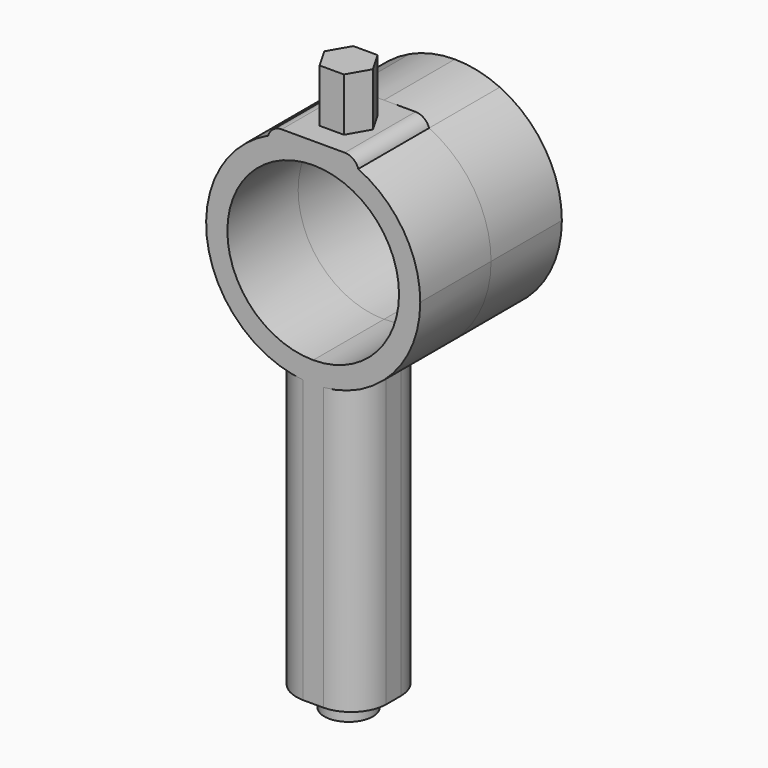
from build123d import *

# Parameters (mm, degrees)
F1_DEPTH     = 12.5
F2_DEPTH     = 12.5
F3_DEPTH     = 12.5
F6_DEPTH     = 7.5
F5_R         = 3.429
F7_DEPTH     = 3
F8_T4_DEPTH  = 66.159380005
F8_S5_R      = 15.125
F8_T6_DEPTH  = 35
F8_T10_DEPTH = 66.159380005
F8_S11_R     = 15.125
F8_T12_DEPTH = 35
F8_T16_DEPTH = 66.159380005
F8_S17_R     = 15.125
F8_T18_DEPTH = 35
F8_T22_DEPTH = 66.159380005
F8_S23_R     = 15.125
F8_T24_DEPTH = 35
F9_T1_DEPTH  = 22.0465191056


# Not quite as in the source:
# - a fillet or chamfer that OpenCascade refuses, or shapes differently, is made with other operations: its cross-section is extruded or revolved along the edge and cut away or added


with BuildPart() as f1:
    # F0 (on Front) → F1 (new body, symmetric)
    with BuildSketch(Plane.XZ):
        with BuildLine():
            Line((-6.3651329838, -12.125), (-6.3651329838, -13.7204485021))
            ThreePointArc((-6.3651329838, -13.7204485021), (0, -15.125), (6.3651329838, -13.7204485021))
            Line((6.3651329838, -13.7204485021), (6.3651329838, -12.125))
            Line((6.3651329838, -12.125), (0, -12.125))
            Line((0, -12.125), (-6.3651329838, -12.125))
        make_face()
        with BuildLine():
            ThreePointArc((6.3651329838, 13.7204485021), (3.2591288258, 14.7696887001), (0, 15.125))
            ThreePointArc((0, 15.125), (-3.2591288258, 14.7696887001), (-6.3651329838, 13.7204485021))
            Line((-6.3651329838, 13.7204485021), (-6.3651329838, 12.125))
            Line((-6.3651329838, 12.125), (0, 12.125))
            Line((0, 12.125), (6.3651329838, 12.125))
            Line((6.3651329838, 12.125), (6.3651329838, 13.7204485021))
        make_face()
        with BuildLine():
            ThreePointArc((15.125, 0), (12.7482991293, 8.1391949424), (6.3651329838, 13.7204485021))
            Line((6.3651329838, 13.7204485021), (6.3651329838, 12.125))
            Line((6.3651329838, 12.125), (0, 12.125))
            ThreePointArc((0, 12.125), (8.5736697219, 8.5736697219), (12.125, 0))
            ThreePointArc((12.125, 0), (8.5736697219, -8.5736697219), (0, -12.125))
            Line((0, -12.125), (6.3651329838, -12.125))
            Line((6.3651329838, -12.125), (6.3651329838, -13.7204485021))
            ThreePointArc((6.3651329838, -13.7204485021), (12.7482991293, -8.1391949424), (15.125, 0))
        make_face()
        with BuildLine():
            Line((-6.3651329838, 12.125), (-6.3651329838, 13.7204485021))
            ThreePointArc((-6.3651329838, 13.7204485021), (-15.125, 0), (-6.3651329838, -13.7204485021))
            Line((-6.3651329838, -13.7204485021), (-6.3651329838, -12.125))
            Line((-6.3651329838, -12.125), (0, -12.125))
            ThreePointArc((0, -12.125), (-12.125, 0), (0, 12.125))
            Line((0, 12.125), (-6.3651329838, 12.125))
        make_face()
    extrude(amount=F1_DEPTH, both=True)

    # F0 (on Front) → F2 (join, through all)
    with BuildSketch(Plane.XZ):
        with BuildLine():
            ThreePointArc((6.3651329838, -13.7204485021), (0, -15.125), (-6.3651329838, -13.7204485021))
            Line((-6.3651329838, -13.7204485021), (-6.3651329838, -54.875))
            Line((-6.3651329838, -54.875), (6.3651329838, -54.875))
            Line((6.3651329838, -54.875), (6.3651329838, -13.7204485021))
        make_face()
    extrude(amount=F2_DEPTH)

    # F0 (on Front) → F3 (join, through all)
    with BuildSketch(Plane.XZ):
        with BuildLine():
            Line((6.3651329838, 15.125), (0, 15.125))
            ThreePointArc((0, 15.125), (3.2591288258, 14.7696887001), (6.3651329838, 13.7204485021))
            Line((6.3651329838, 13.7204485021), (6.3651329838, 15.125))
        make_face()
        with BuildLine():
            Line((0, 15.125), (-6.3651329838, 15.125))
            Line((-6.3651329838, 15.125), (-6.3651329838, 13.7204485021))
            ThreePointArc((-6.3651329838, 13.7204485021), (-3.2591288258, 14.7696887001), (0, 15.125))
        make_face()
    extrude(amount=F3_DEPTH)

    # F4 (on face) → F6 (join)
    with BuildSketch(Plane.XY.offset(15.125)):
        Polygon((1.7145000001, -9.2196011096), (3.4290000001, -6.25), (1.7144999999, -3.2803988905), (-1.7145, -3.2803988907), (-3.4289999999, -6.25), (-1.7145000001, -9.2196011096), align=None)
    extrude(amount=F6_DEPTH)

    # F5 (on face) → F7 (join)
    with BuildSketch(Plane(origin=(0, 0, -54.875), x_dir=(1, 0, 0), z_dir=(0, 0, -1))):
        with Locations((0, 6.2500000003)):
            Circle(F5_R)
    extrude(amount=F7_DEPTH)

    # F8: fillet of radius 5 on 6 edges, made by hand


with BuildPart() as f8_tool2:
    # F8_s3 → F8_t4 (new body)
    with BuildSketch(Plane.XY.offset(-67.3774142536)):
        with BuildLine():
            ThreePointArc((1.3641672983, 0.0004), (4.9006668897, -1.4644660941), (6.3655329838, -5.0009656854))
            Line((6.3655329838, -5.0009656854), (6.8656695523, -5.0009656854))
            ThreePointArc((6.8656695523, -5.0009656854), (6.8652695523, -2.5004828427), (6.8652695523, 0))
            Line((6.8652695523, 0), (6.3651329838, 0.5001365685))
            ThreePointArc((6.3651329838, 0.5001365685), (3.8646501411, 0.5001365685), (1.3641672983, 0.5005365685))
            Line((1.3641672983, 0.5005365685), (1.3641672983, 0.0004))
        make_face()
    extrude(amount=F8_T4_DEPTH)

    # F8_s5 → F8_t6 (cut, symmetric)
    with BuildSketch(Plane.XZ.offset(2.3)):
        Circle(F8_S5_R)
    extrude(amount=F8_T6_DEPTH, both=True, mode=Mode.SUBTRACT)


with BuildPart() as f1_1:
    add(f1.part)

    # F8_t1: cut F8_tool2
    add(f8_tool2.part, mode=Mode.SUBTRACT)


with BuildPart() as f8_tool8:
    # F8_s9 → F8_t10 (new body)
    with BuildSketch(Plane.XY.offset(-1.2180342485)):
        with BuildLine():
            ThreePointArc((-6.3655329838, -5.0009656854), (-4.9006668897, -1.4644660941), (-1.3641672983, 0.0004))
            Line((-1.3641672983, 0.0004), (-1.3641672983, 0.5005365685))
            ThreePointArc((-1.3641672983, 0.5005365685), (-3.8646501411, 0.5001365685), (-6.3651329838, 0.5001365685))
            Line((-6.3651329838, 0.5001365685), (-6.8652695523, 0))
            ThreePointArc((-6.8652695523, 0), (-6.8652695523, -2.5004828427), (-6.8656695523, -5.0009656854))
            Line((-6.8656695523, -5.0009656854), (-6.3655329838, -5.0009656854))
        make_face()
    extrude(amount=-F8_T10_DEPTH)

    # F8_s11 → F8_t12 (cut, symmetric)
    with BuildSketch(Plane.XZ.offset(2.3)):
        Circle(F8_S11_R)
    extrude(amount=F8_T12_DEPTH, both=True, mode=Mode.SUBTRACT)


with BuildPart() as f1_2:
    add(f1_1.part)

    # F8_t7: cut F8_tool8
    add(f8_tool8.part, mode=Mode.SUBTRACT)


with BuildPart() as f8_tool14:
    # F8_s15 → F8_t16 (new body)
    with BuildSketch(Plane.XY.offset(-67.3774142536)):
        with BuildLine():
            ThreePointArc((1.3641672983, -12.5004), (4.9006668897, -11.0355339059), (6.3655329838, -7.4990343146))
            Line((6.3655329838, -7.4990343146), (6.8656695523, -7.4990343146))
            ThreePointArc((6.8656695523, -7.4990343146), (6.8652695523, -9.9995171573), (6.8652695523, -12.5))
            Line((6.8652695523, -12.5), (6.3651329838, -13.0001365685))
            ThreePointArc((6.3651329838, -13.0001365685), (3.8646501411, -13.0001365685), (1.3641672983, -13.0005365685))
            Line((1.3641672983, -13.0005365685), (1.3641672983, -12.5004))
        make_face()
    extrude(amount=F8_T16_DEPTH)

    # F8_s17 → F8_t18 (cut, symmetric)
    with BuildSketch(Plane.XZ.offset(10.2)):
        Circle(F8_S17_R)
    extrude(amount=F8_T18_DEPTH, both=True, mode=Mode.SUBTRACT)


with BuildPart() as f1_3:
    add(f1_2.part)

    # F8_t13: cut F8_tool14
    add(f8_tool14.part, mode=Mode.SUBTRACT)


with BuildPart() as f8_tool20:
    # F8_s21 → F8_t22 (new body)
    with BuildSketch(Plane.XY.offset(-1.2180342485)):
        with BuildLine():
            ThreePointArc((-1.3641672983, -12.5004), (-4.9006668897, -11.0355339059), (-6.3655329838, -7.4990343146))
            Line((-6.3655329838, -7.4990343146), (-6.8656695523, -7.4990343146))
            ThreePointArc((-6.8656695523, -7.4990343146), (-6.8652695523, -9.9995171573), (-6.8652695523, -12.5))
            Line((-6.8652695523, -12.5), (-6.3651329838, -13.0001365685))
            ThreePointArc((-6.3651329838, -13.0001365685), (-3.8646501411, -13.0001365685), (-1.3641672983, -13.0005365685))
            Line((-1.3641672983, -13.0005365685), (-1.3641672983, -12.5004))
        make_face()
    extrude(amount=-F8_T22_DEPTH)

    # F8_s23 → F8_t24 (cut, symmetric)
    with BuildSketch(Plane.XZ.offset(10.2)):
        Circle(F8_S23_R)
    extrude(amount=F8_T24_DEPTH, both=True, mode=Mode.SUBTRACT)


with BuildPart() as f1_4:
    add(f1_3.part)

    # F8_t19: cut F8_tool20
    add(f8_tool20.part, mode=Mode.SUBTRACT)

    # F9: fillet of radius 2 on 2 edges, made by hand

    # F9_s2 → F9_t1 (cut)
    with BuildSketch(Plane.XZ.offset(-4.7732595528)):
        with BuildLine():
            ThreePointArc((-6.3651329838, 13.7204485021), (-5.6409669175, 14.7360395719), (-4.4558291627, 15.125))
            Line((-4.4558291627, 15.125), (-6.3651329838, 15.125))
            Line((-6.3651329838, 15.125), (-6.3651329838, 13.7204485021))
        make_face()
        with BuildLine():
            ThreePointArc((4.4558291627, 15.125), (5.6409669175, 14.7360395719), (6.3651329838, 13.7204485021))
            Line((6.3651329838, 13.7204485021), (6.3651329838, 15.125))
            Line((6.3651329838, 15.125), (4.4558291627, 15.125))
        make_face()
    extrude(amount=F9_T1_DEPTH, mode=Mode.SUBTRACT)


solid = f1_4.part
